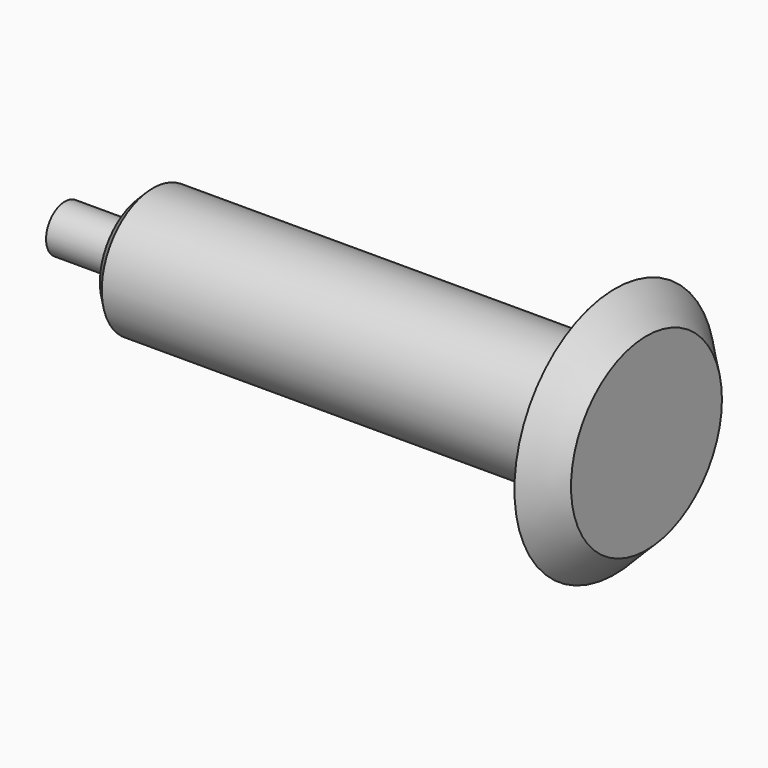
from build123d import *

# Parameters (mm, degrees)
F0_W     = 25
F0_H     = 7.5
F2_SIZE2 = 3
F2_SIZE  = 3
F3_SIZE2 = 9.99999
F3_SIZE  = 9.99999
F4_SIZE2 = 9.99999
F4_SIZE  = 9.99999


# Not quite as in the source:
# - a fillet or chamfer is up to 0.001 mm smaller than in the source, because OpenCascade refuses the exact size


with BuildPart() as f1:
    # F0 (on Top) → F1 (revolve)
    with BuildSketch(Plane.XY):
        with Locations((-12.5, 3.75)):
            Rectangle(F0_W, F0_H)
        Polygon((0, 7.5), (0, 0), (140, 0), (140, 20.3452128917), (0, 20.3452128917), align=None)
        Polygon((140, 20.3452128917), (140, 0), (150, 0), (150, 30.6925382465), (140, 30.6925382465), align=None)
        Polygon((150, 30.6925382465), (150, 0), (160, 0), (160, 40), (150, 40), align=None)
    revolve(axis=Axis((70, 0, 0), (1, 0, 0)))

    # F2
    f2_edges = [f1.edges().sort_by_distance(p)[0] for p in [
        (0, -20.345213, 0),
    ]]
    chamfer(f2_edges, length=F2_SIZE, length2=F2_SIZE2)

    # F3 (size 10 and 10 in the source; OpenCascade refuses exactly that, so slightly less here)
    f3_edges = [f1.edges().sort_by_distance(p)[0] for p in [
        (140, -30.692538, 0),
    ]]
    chamfer(f3_edges, length=F3_SIZE, length2=F3_SIZE2)

    # F4 (size 10 and 10 in the source; OpenCascade refuses exactly that, so slightly less here)
    f4_edges = [f1.edges().sort_by_distance(p)[0] for p in [
        (160, -40, 0),
    ]]
    chamfer(f4_edges, length=F4_SIZE, length2=F4_SIZE2)


solid = f1.part
